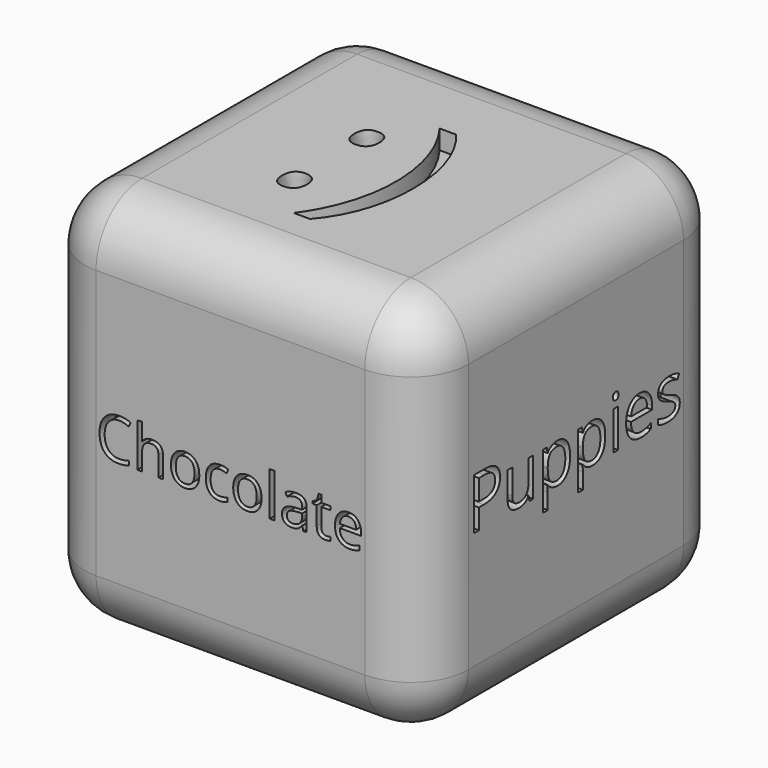
from build123d import *

# Parameters (mm, degrees)
F0_W         = 25.4
F0_H         = 25.4
F1_DEPTH     = 25.4
F2_R         = 3.81
F8_TEXT_SIZE = 13.8601301134
F9_DEPTH     = 1.27
F3_TEXT_SIZE = 5.5448786668
F10_DEPTH    = 1.27
F5_TEXT_SIZE = 4.32209055
F11_DEPTH    = 1.27
F4_TEXT_SIZE = 4.7395559998
F12_DEPTH    = 1.27
F6_TEXT_SIZE = 3.8117442133
F13_DEPTH    = 1.27
F7_TEXT_SIZE = 4.2009820209
F14_DEPTH    = 1.27


# Not quite as in the source:
# - Text() gives the source's letters only with a copy of the font that has no kerning and outlines rounded to 1/6400 em; it was checked with that copy


with BuildPart() as f1:
    # F0 (on Top) → F1 (new body)
    with BuildSketch(Plane.XY):
        with Locations((-12.7, 12.7)):
            Rectangle(F0_W, F0_H)
    extrude(amount=F1_DEPTH)

    # F2
    f2_edges = [f1.edges().sort_by_distance(p)[0] for p in [
        (-12.7, 0, 25.4),
        (0, 12.7, 25.4),
        (-12.7, 25.4, 25.4),
        (-25.4, 12.7, 25.4),
        (-12.7, 0, 0),
        (0, 0, 12.7),
        (0, 12.7, 0),
        (0, 25.4, 12.7),
        (-25.4, 0, 12.7),
        (-25.4, 12.7, 0),
        (-25.4, 25.4, 12.7),
        (-12.7, 25.4, 0),
    ]]
    fillet(f2_edges, radius=F2_R)

    # F8 (on face) → F9 (cut)
    with BuildSketch(Plane.XY.offset(25.4)):
        with Locations((-17.1731822193, 7.8716045246)):
            Text(':)', F8_TEXT_SIZE, font='Open Sans', text_align=(TextAlign.LEFT, TextAlign.BOTTOM))
    extrude(amount=-F9_DEPTH, mode=Mode.SUBTRACT)

    # F3 (on face) → F10 (cut)
    with BuildSketch(Plane(origin=(0, 25.4, 0), x_dir=(-1, 0, 0), z_dir=(0, 1, 0))):
        with Locations((3.81, 10.9175111303)):
            Text('People', F3_TEXT_SIZE, font='Open Sans', text_align=(TextAlign.LEFT, TextAlign.BOTTOM))
    extrude(amount=-F10_DEPTH, mode=Mode.SUBTRACT)

    # F5 (on face) → F11 (cut)
    with BuildSketch(Plane(origin=(-25.4, 0, 0), x_dir=(0, -1, 0), z_dir=(-1, 0, 0))):
        with Locations((-21.59, 11.3795931261)):
            Text('Learning', F5_TEXT_SIZE, font='Open Sans', text_align=(TextAlign.LEFT, TextAlign.BOTTOM))
    extrude(amount=-F11_DEPTH, mode=Mode.SUBTRACT)

    # F4 (on face) → F12 (cut)
    with BuildSketch(Plane.YZ):
        with Locations((3.81, 11.5734190236)):
            Text('Puppies', F4_TEXT_SIZE, font='Open Sans', text_align=(TextAlign.LEFT, TextAlign.BOTTOM))
    extrude(amount=-F12_DEPTH, mode=Mode.SUBTRACT)

    # F6 (on face) → F13 (cut)
    with BuildSketch(Plane.XZ):
        with Locations((-21.59, 10.8619248455)):
            Text('Chocolate', F6_TEXT_SIZE, font='Open Sans', text_align=(TextAlign.LEFT, TextAlign.BOTTOM))
    extrude(amount=-F13_DEPTH, mode=Mode.SUBTRACT)

    # F7 (on face) → F14 (cut)
    with BuildSketch(Plane(origin=(0, 0, 0), x_dir=(1, 0, 0), z_dir=(0, 0, -1))):
        with Locations((-21.59, -14.3710090687)):
            Text('Listening', F7_TEXT_SIZE, font='Open Sans', text_align=(TextAlign.LEFT, TextAlign.BOTTOM))
    extrude(amount=-F14_DEPTH, mode=Mode.SUBTRACT)


solid = f1.part
